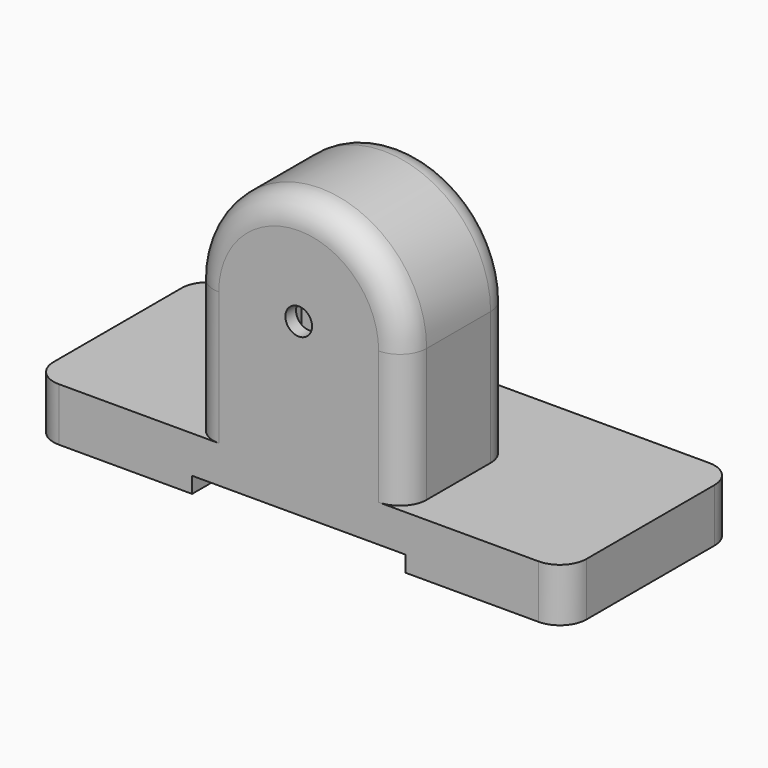
from build123d import *

# Parameters (mm, degrees)
F0_W      = 100
F0_H      = 40
F1_DEPTH  = 10
F3_R      = 5
F4_R      = 5
F5_R      = 5
F6_R      = 5
F7_DEPTH  = 25
F8_T      = -2.5
F9_R      = 5
F10_R     = 5
F12_D     = 5
F13_W     = 40
F13_H     = 3
F14_DEPTH = 40.001


# Not quite as in the source:
# - a shell that OpenCascade refuses in one call is made with other operations: the cavity is built on its own and cut out


with BuildPart() as f1:
    # F0 (on Top) → F1 (new body)
    with BuildSketch(Plane.XY):
        with Locations((50, -20)):
            Rectangle(F0_W, F0_H)
    extrude(amount=F1_DEPTH)

    # F3
    f3_edges = [f1.edges().sort_by_distance(p)[0] for p in [
        (100, -40, 5),
    ]]
    fillet(f3_edges, radius=F3_R)

    # F4
    f4_edges = [f1.edges().sort_by_distance(p)[0] for p in [
        (100, 0, 5),
    ]]
    fillet(f4_edges, radius=F4_R)

    # F5
    f5_edges = [f1.edges().sort_by_distance(p)[0] for p in [
        (0, -40, 5),
    ]]
    fillet(f5_edges, radius=F5_R)

    # F6
    f6_edges = [f1.edges().sort_by_distance(p)[0] for p in [
        (0, 0, 5),
    ]]
    fillet(f6_edges, radius=F6_R)

    # F2 (on face) → F7 (join)
    with BuildSketch(Plane.XZ.offset(40)):
        with BuildLine():
            Line((30, 35), (30, 10))
            Line((30, 10), (70, 10))
            Line((70, 10), (70, 35))
            ThreePointArc((70, 35), (50, 55), (30, 35))
        make_face()
    extrude(amount=-F7_DEPTH)

    # F8: a shell. OpenCascade refuses it in one call, so the cavity is built on its own and cut out:
    # the body offset inwards by the wall thickness, plus a prism from it out through each open face.
    f8_core = offset(f1.part, amount=F8_T, kind=Kind.INTERSECTION, mode=Mode.PRIVATE)
    f8_exits = [f8_core.faces().sort_by_distance(p)[0] for p in [
        (50, -2.5, 5),
    ]]
    add(f8_core, mode=Mode.SUBTRACT)
    extrude(f8_exits, amount=-F8_T, mode=Mode.SUBTRACT)

    # F9
    f9_edges = [f1.edges().sort_by_distance(p)[0] for p in [
        (30, -40, 22.5),
    ]]
    fillet(f9_edges, radius=F9_R)

    # F10
    f10_edges = [f1.edges().sort_by_distance(p)[0] for p in [
        (30, -15, 22.5),
    ]]
    fillet(f10_edges, radius=F10_R)

    # F12 (through all)
    with Locations(Plane.XZ.offset(40)):
        with Locations((50, 35)):
            Hole(F12_D / 2)

    # F13 (on face) → F14 (cut, through all)
    with BuildSketch(Plane.XZ.offset(40)):
        with Locations((50, 1.5)):
            Rectangle(F13_W, F13_H)
    extrude(amount=-F14_DEPTH, mode=Mode.SUBTRACT)


solid = f1.part
